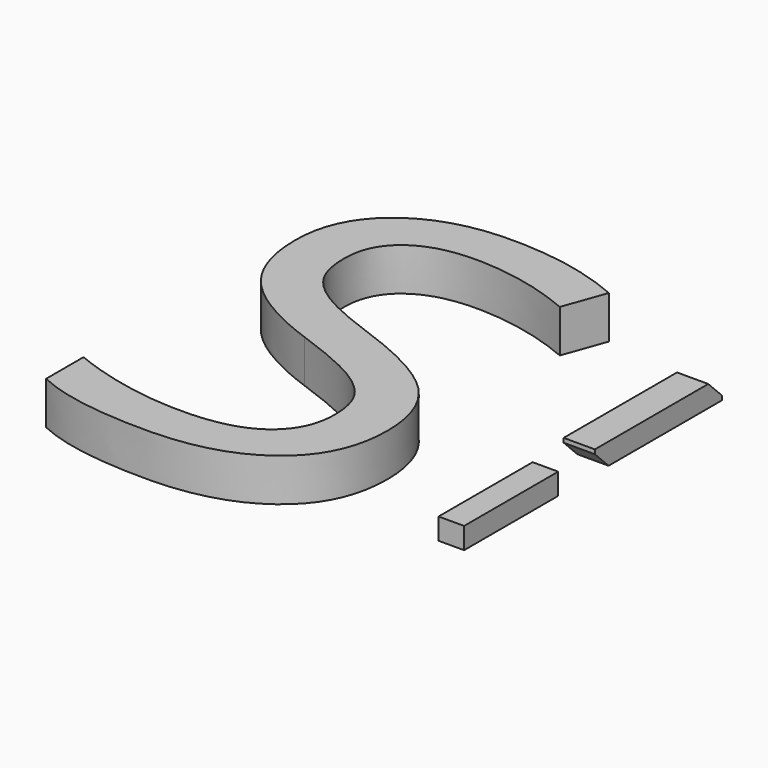
from build123d import *

# Parameters (mm, degrees)
F1_W         = 9.2769190669
F1_H         = 47.1576601267
F2_DEPTH     = 6.35
F3_SIZE      = 5.08
F4_SIZE      = 5.08
F0_TEXT_SIZE = 173.9421859384
F5_DEPTH     = 12.7
F6_W         = 7.5919553638
F6_H         = 34.9229648709
F7_DEPTH     = 6.35


# Not quite as in the source:
# - Text() gives the source's letters only with a copy of the font that has no kerning and outlines rounded to 1/6400 em; it was checked with that copy


with BuildPart() as f2:
    # F1 (on Top) → F2 (new body)
    with BuildSketch(Plane.XY):
        with Locations((61.2663067877, 23.5788300633)):
            Rectangle(F1_W, F1_H)
    extrude(amount=F2_DEPTH)

    # F3
    f3_edges = [f2.edges().sort_by_distance(p)[0] for p in [
        (61.266307, 47.15766, 6.35),
    ]]
    chamfer(f3_edges, length=F3_SIZE)

    # F4
    f4_edges = [f2.edges().sort_by_distance(p)[0] for p in [
        (61.266307, 0, 0),
    ]]
    chamfer(f4_edges, length=F4_SIZE)


with BuildPart() as f5:
    # F0 (on Top) → F5 (new body)
    with BuildSketch(Plane.XY):
        with Locations((-57.0143833756, -65.324947238)):
            Text('S', F0_TEXT_SIZE, font='Open Sans', text_align=(TextAlign.LEFT, TextAlign.BOTTOM))
    extrude(amount=F5_DEPTH)


with BuildPart() as f7:
    # F6 (on Top) → F7 (new body)
    with BuildSketch(Plane.XY):
        with Locations((62.4437704682, -31.5065868199)):
            Rectangle(F6_W, F6_H)
    extrude(amount=F7_DEPTH)


solid = Compound([f2.part, f5.part, f7.part])
